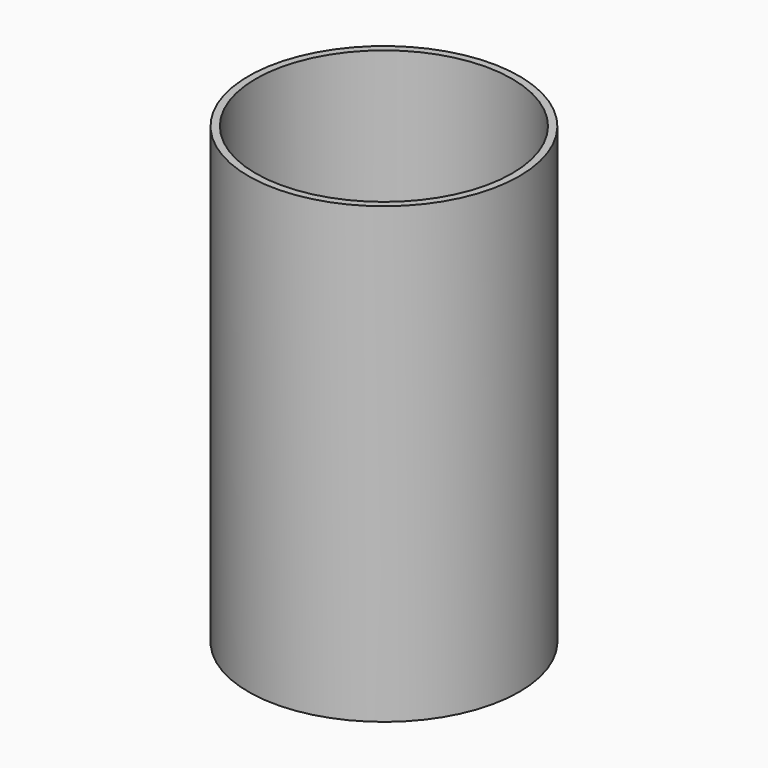
from build123d import *

# Parameters (mm, degrees)
F0_R     = 46.99
F0_R_2   = 44.45
F1_DEPTH = 152.4
F2_R     = 46.99
F2_R_2   = 44.45
F3_DEPTH = 5.08


with BuildPart() as f1:
    # F0 (on Top) → F1 (new body)
    with BuildSketch(Plane.XY):
        Circle(F0_R)
        Circle(F0_R_2, mode=Mode.SUBTRACT)
    extrude(amount=F1_DEPTH)

    # F2 (on face) → F3 (join)
    with BuildSketch(Plane(origin=(0, 0, 0), x_dir=(1, 0, 0), z_dir=(0, 0, -1))):
        Circle(F2_R)
        Circle(F2_R_2, mode=Mode.SUBTRACT)
        Circle(F2_R_2)
    extrude(amount=F3_DEPTH)


solid = f1.part
